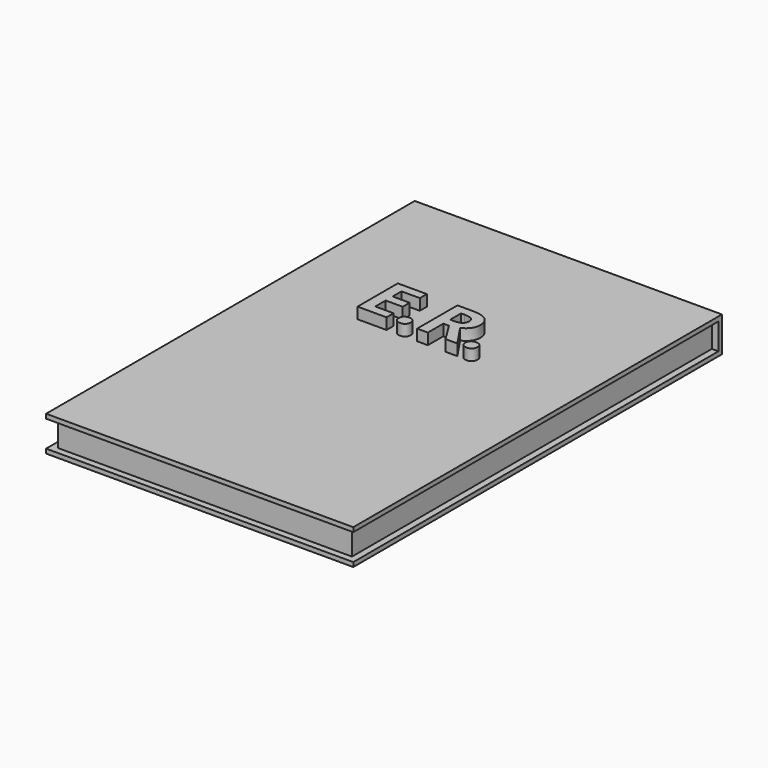
from build123d import *

# Parameters (mm, degrees)
F0_W         = 140
F0_H         = 210
F1_DEPTH     = 16
F2_W         = 208
F2_H         = 12
F5_DEPTH     = 3
F4_W         = 140
F4_H         = 12
F6_DEPTH     = 3
F3_W         = 208
F3_H         = 12
F7_DEPTH     = 3
F8_TEXT_SIZE = 32.1364651124
F9_DEPTH     = 5.08


# Not quite as in the source:
# - Text() gives the source's letters only with a copy of the font that has no kerning and outlines rounded to 1/6400 em; it was checked with that copy


with BuildPart() as f1:
    # F0 (on Top) → F1 (new body)
    with BuildSketch(Plane.XY):
        with Locations((6.4437575638, -21.0727320282)):
            Rectangle(F0_W, F0_H)
    extrude(amount=F1_DEPTH)

    # F2 (on face) → F5 (cut)
    with BuildSketch(Plane.YZ.offset(76.4437575638)):
        with Locations((-22.0727320282, 8)):
            Rectangle(F2_W, F2_H)
    extrude(amount=-F5_DEPTH, mode=Mode.SUBTRACT)

    # F4 (on face) → F6 (cut)
    with BuildSketch(Plane.XZ.offset(126.0727320282)):
        with Locations((6.4437575638, 8)):
            Rectangle(F4_W, F4_H)
    extrude(amount=-F6_DEPTH, mode=Mode.SUBTRACT)

    # F3 (on face) → F7 (cut)
    with BuildSketch(Plane(origin=(-63.5562424362, 0, 0), x_dir=(0, -1, 0), z_dir=(-1, 0, 0))):
        with Locations((22.0727320282, 8)):
            Rectangle(F3_W, F3_H)
    extrude(amount=-F7_DEPTH, mode=Mode.SUBTRACT)

    # F8 (on face) → F9 (join)
    with BuildSketch(Plane.XY.offset(16)):
        with Locations((-25.360757485, 0)):
            Text('E.R.', F8_TEXT_SIZE, font='Open Sans', font_style=FontStyle.BOLD, text_align=(TextAlign.LEFT, TextAlign.BOTTOM))
    extrude(amount=F9_DEPTH)


solid = f1.part
